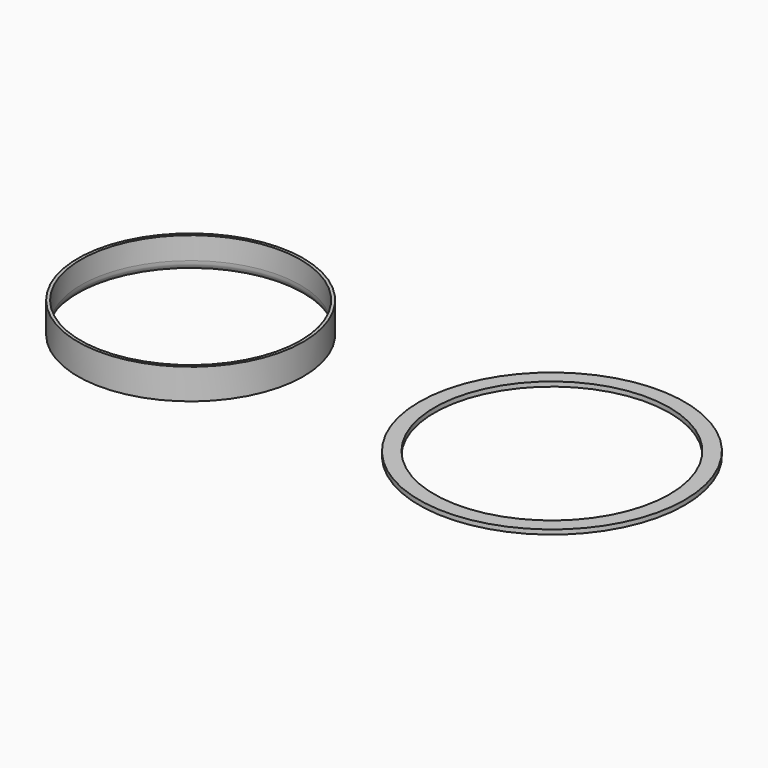
from build123d import *

# Parameters (mm, degrees)
F1_R     = 43.6066034391
F1_R_2   = 38.6066034391
F2_DEPTH = 1.5
F0_R     = 37.0683102398
F0_R_2   = 36.0578095469
F3_DEPTH = 10


# Not quite as in the source:
# - a fillet or chamfer that OpenCascade refuses, or shapes differently, is made with other operations: its cross-section is extruded or revolved along the edge and cut away or added
# - a feature names something its author has since deleted; it is built from what else it names


with BuildPart() as f2:
    # F1 (on Top) → F2 (new body)
    with BuildSketch(Plane.XY):
        Circle(F1_R)
        Circle(F1_R_2, mode=Mode.SUBTRACT)
    extrude(amount=F2_DEPTH)


with BuildPart() as f3:
    # F0 (on Top) → F3 (new body)
    with BuildSketch(Plane.XY):
        with Locations((-114.4955381751, -5.2098422311)):
            Circle(F0_R)
        with Locations((-114.4955381751, -5.2098422311)):
            Circle(F0_R_2, mode=Mode.SUBTRACT)
    extrude(amount=F3_DEPTH)

    # F5: fillet of radius 4 on 1 edges, made by hand

    # F5_s1 → F5_t2 (revolve, cut)
    with BuildSketch(Plane.XZ.offset(5.2098422311)):
        with BuildLine():
            ThreePointArc((-78.4377286282, 2.6576105607), (-78.1765785335, 1.2359912778), (-77.4272279353, 0))
            Line((-77.4272279353, 0), (-78.4377286282, 0))
            Line((-78.4377286282, 0), (-78.4377286282, 2.6576105607))
        make_face()
    revolve(axis=Axis((-114.4955381751, -5.2098422311, 0), (0, 0, 1)), mode=Mode.SUBTRACT)


solid = Compound([f2.part, f3.part])
